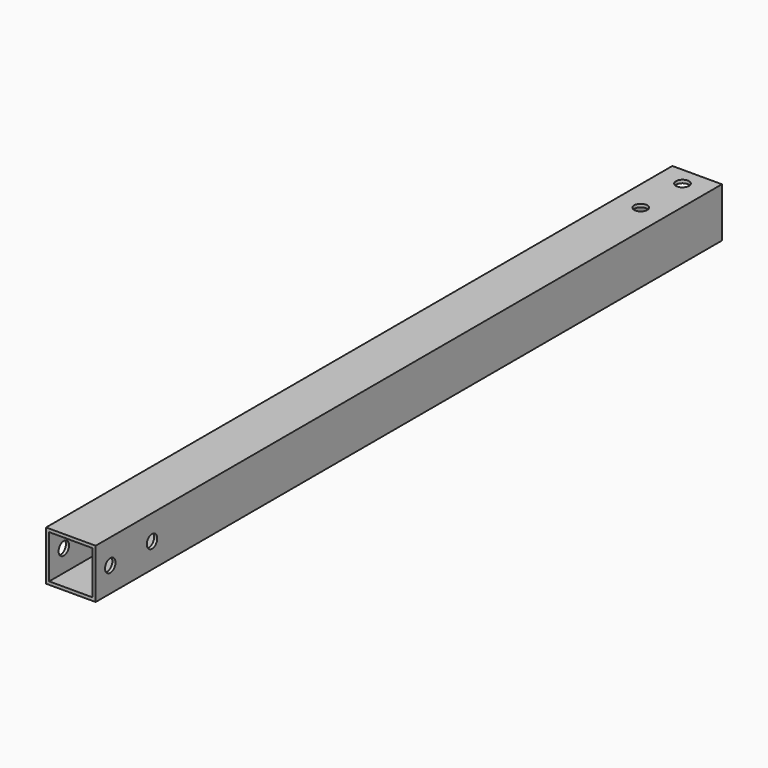
from build123d import *

# Parameters (mm, degrees)
F1_W       = 19
F1_H       = 19
F1_W_2     = 16.6
F1_H_2     = 16.6
F2_DEPTH   = 300
F5_D       = 5
F5_ON_F4_D = 5


# Not quite as in the source:
# - a feature names something its author has since deleted; it is built from what else it names


with BuildPart() as f2:
    # F1 (on Front) → F2 (new body)
    with BuildSketch(Plane.XZ):
        Rectangle(F1_W, F1_H)
        Rectangle(F1_W_2, F1_H_2, mode=Mode.SUBTRACT)
    extrude(amount=-F2_DEPTH)

    # F5 (through all)
    with Locations(Plane.YZ.offset(9.5)):
        with Locations((7, 0), (27, 0)):
            Hole(F5_D / 2)

    # F5 on F4 (through all)
    with Locations(Plane.XY.offset(9.5)):
        with Locations((0, 273), (0, 293)):
            Hole(F5_ON_F4_D / 2)


solid = f2.part
